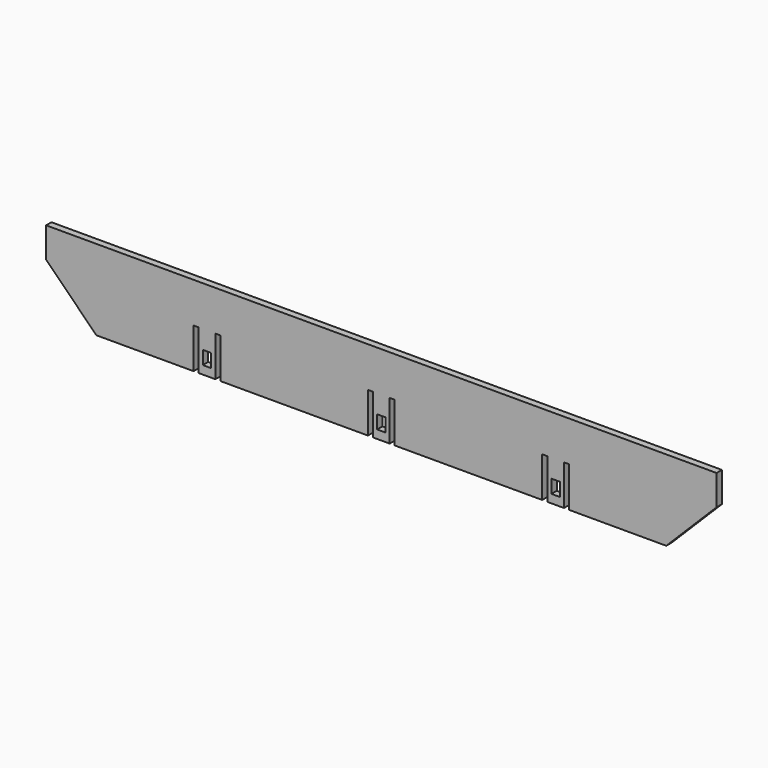
from build123d import *

# Parameters (mm, degrees)
F0_W     = 2.5
F0_H     = 4
F1_DEPTH = 2


# Not quite as in the source:
# - a feature names something its author has since deleted; it is built from what else it names


with BuildPart() as f1:
    # F0 (on Front) → F1 (new body)
    with BuildSketch(Plane.XZ):
        Polygon((56, -7.5), (85, -7.5), (85, 7.5), (-85, 7.5), (-85, -7.5), (-56, -7.5), (-56, 4.5), (-54.5, 4.5), (-54.5, -7.5), (-49.5, -7.5), (-49.5, 4.5), (-48, 4.5), (-48, -7.5), (-4, -7.5), (-4, 4.5), (-2.5, 4.5), (-2.5, -7.5), (2.5, -7.5), (2.5, 4.5), (4, 4.5), (4, -7.5), (48, -7.5), (48, 4.5), (49.5, 4.5), (49.5, -7.5), (54.5, -7.5), (54.5, 4.5), (56, 4.5), align=None)
        with Locations((-52, -3)):
            Rectangle(F0_W, F0_H, mode=Mode.SUBTRACT)
        with Locations((0, -3)):
            Rectangle(F0_W, F0_H, mode=Mode.SUBTRACT)
        with Locations((52, -3)):
            Rectangle(F0_W, F0_H, mode=Mode.SUBTRACT)
        Polygon((-85, -7.5), (-85, 7.5), (-100, 7.5), align=None)
        Polygon((85, 7.5), (85, -7.5), (100, 7.5), align=None)
        Polygon((-85, 7.5), (85, 7.5), (100, 7.5), (100, 16.5), (-100, 16.5), (-100, 7.5), align=None)
    extrude(amount=F1_DEPTH)


solid = f1.part
